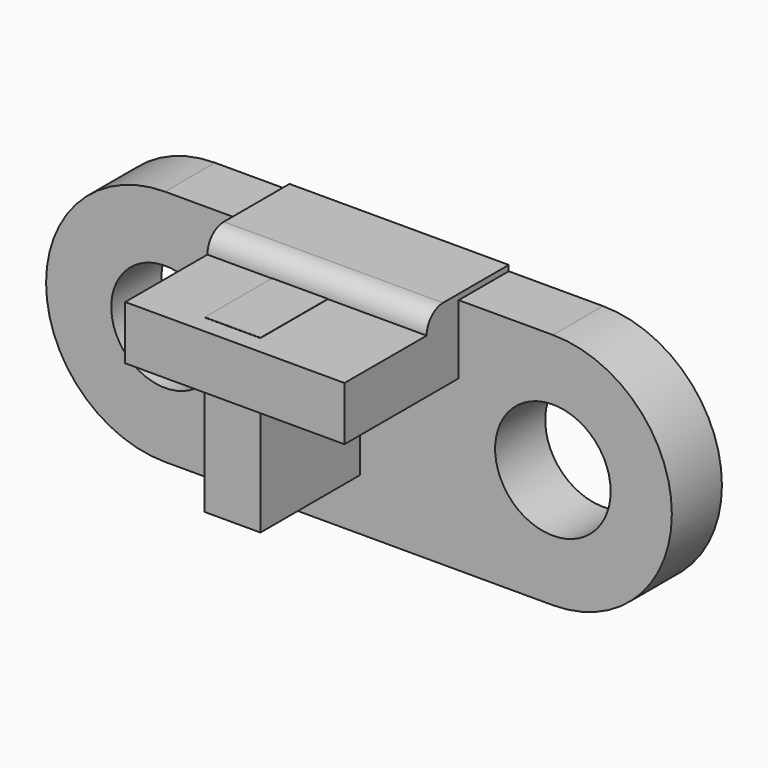
from build123d import *

# Parameters (mm, degrees)
F0_R     = 13.3135020733
F0_R_2   = 14.2906457186
F1_DEPTH = 15.4849458486
F2_W     = 54.254218936
F2_H     = 18.4195190668
F3_DEPTH = 25.4
F4_R     = 5.08
F5_DEPTH = 25.4
F6_W     = 46.2679080665
F6_H     = 42.419552803
F7_DEPTH = 13.794451952


# Not quite as in the source:
# - the program builds the solid bodies; features that only make, move or delete a surface that nothing else refers to are left out


with BuildPart() as f1:
    # F0 (on Front) → F1 (new body)
    with BuildSketch(Plane.XZ):
        with BuildLine():
            Line((47.7382689714, 29.4530540705), (-48.2266321778, 29.4530540705))
            ThreePointArc((-48.2266321778, 29.4530540705), (-77.6628926396, 0.0167936087), (-48.2266321778, -29.4194668531))
            Line((-48.2266321778, -29.4194668531), (47.7382689714, -29.4194668531))
            ThreePointArc((47.7382689714, -29.4194668531), (77.1745294333, 0.0167936087), (47.7382689714, 29.4530540705))
        make_face()
        with Locations((-48.2266321778, 0.0167936087)):
            Circle(F0_R, mode=Mode.SUBTRACT)
        with Locations((47.7382689714, 0.0167936087)):
            Circle(F0_R_2, mode=Mode.SUBTRACT)
    extrude(amount=F1_DEPTH)

    # F2 (on Front) → F3 (join)
    with BuildSketch(Plane.XZ):
        with Locations((-2.6991143823, 21.6291323304)):
            Rectangle(F2_W, F2_H)
    extrude(amount=F3_DEPTH)

    # F4
    f4_edges = [f1.edges().sort_by_distance(p)[0] for p in [
        (-2.699114, -25.4, 30.838892),
    ]]
    fillet(f4_edges, radius=F4_R)

    # F5 (add): a face of the model
    f5_faces = [f1.faces().sort_by_distance(p)[0] for p in [
        (-2.6991143823, -25.4, 19.0891323304),
    ]]
    extrude(f5_faces, amount=F5_DEPTH)

    # F6 (on Right) → F7 (join)
    with BuildSketch(Plane.YZ):
        with Locations((-23.1339540333, 4.6068131924)):
            Rectangle(F6_W, F6_H)
    extrude(amount=-F7_DEPTH)


solid = f1.part
